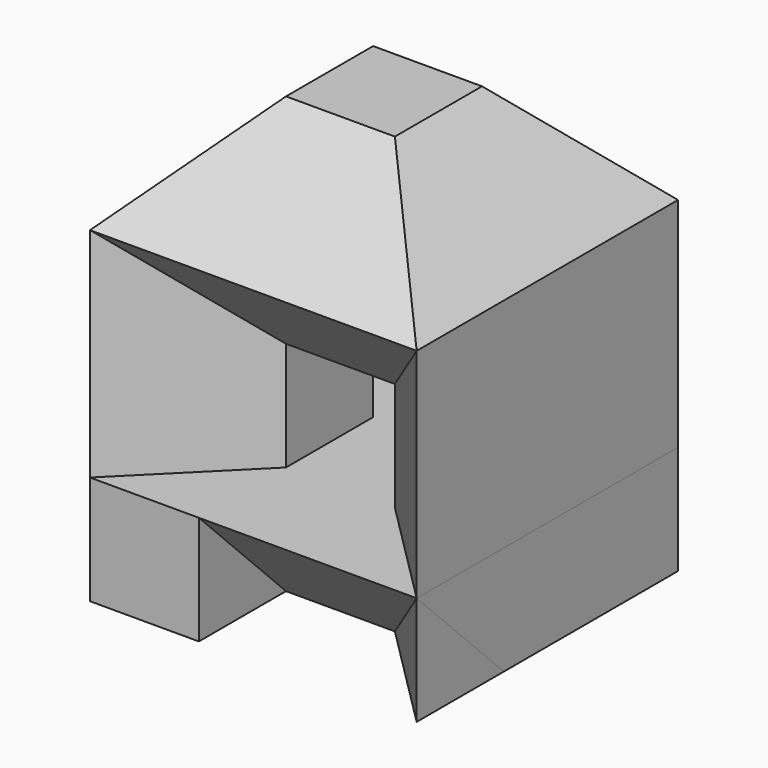
from build123d import *

# Parameters (mm, degrees)
F5_W      = 75
F5_H      = 75
F6_W      = 25
F6_H      = 25
F8_W      = 25
F8_H      = 25
F11_REACH = 179.0579416042
F13_REACH = 179.0579416042
F0_W      = 75
F0_H      = 75
F14_DEPTH = 25
F16_START = 25
F16_DEPTH = 50


with BuildPart() as f7:
    # F5 (on offset) → F7 section 0
    with BuildSketch(Plane.XY.offset(75)):
        with Locations((37.5, 37.5)):
            Rectangle(F5_W, F5_H)
    # F6 (on offset) → F7 section 1
    with BuildSketch(Plane.XY.offset(100)):
        with Locations((37.5, 37.5)):
            Rectangle(F6_W, F6_H)
    loft()


with BuildPart() as f9:
    # F5 (on offset) → F9 section 0
    with BuildSketch(Plane.XY.offset(75)):
        with Locations((37.5, 37.5)):
            Rectangle(F5_W, F5_H)
    # F8 (on offset) → F9 section 1
    with BuildSketch(Plane.XY.offset(50)):
        with Locations((37.5, 37.5)):
            Rectangle(F8_W, F8_H)
    loft()

    f11_end = f9.faces().sort_by_distance((64.5833333333, 37.5, 64.5833333333))[0]
    # F10 (on Top) → F11 (join, up to a face of the model that its end follows)
    with BuildSketch(Plane.XY):
        Polygon((50, 25), (75, 0), (75, 75), (50, 50), align=None)
    f11_long = extrude(amount=F11_REACH, mode=Mode.PRIVATE)
    add(split(f11_long, bisect_by=f11_end, keep=Keep.TOP, mode=Mode.PRIVATE))


with BuildPart() as f13:
    f13_end = f9.part.faces().sort_by_distance((10.4166666667, 37.5, 64.5833333333))[0]
    # F12 (on Top) → F13 (new body, up to a face of F9 that its end follows)
    with BuildSketch(Plane.XY):
        Polygon((25, 50), (0, 75), (0, 0), (25, 25), align=None)
    f13_long = extrude(amount=F13_REACH, mode=Mode.PRIVATE)
    add(split(f13_long, bisect_by=f13_end, keep=Keep.TOP, mode=Mode.PRIVATE))


with BuildPart() as f14:
    # F0 (on Top) → F14 (new body)
    with BuildSketch(Plane.XY):
        with Locations((37.5, 37.5)):
            Rectangle(F0_W, F0_H)
    extrude(amount=F14_DEPTH)

    # F15 (on Right) → F16 (cut)
    with BuildSketch(Plane.YZ.offset(F16_START)):
        Polygon((25, 0), (0, 25), (0, 0), align=None)
    extrude(amount=F16_DEPTH, mode=Mode.SUBTRACT)


solid = Compound([f7.part, f9.part, f13.part, f14.part])
